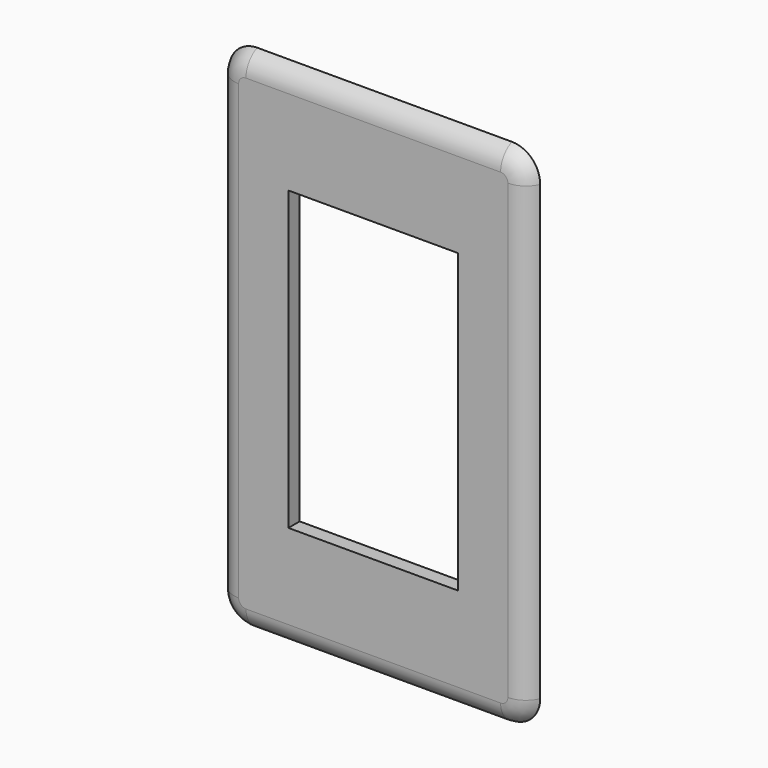
from build123d import *

# Parameters (mm, degrees)
F0_W         = 38.1
F0_H         = 66.675
F1_DEPTH     = 3.175
F2_T1_DEPTH  = 57.15
F2_T3_DEPTH  = 101.6
F2_T6_ANGLE  = 90
F2_T8_ANGLE  = 90
F2_T10_ANGLE = 90
F2_T12_ANGLE = 90


# Not quite as in the source:
# - a fillet or chamfer that OpenCascade refuses, or shapes differently, is made with other operations: its cross-section is extruded or revolved along the edge and cut away or added


with BuildPart() as f1:
    # F0 (on Front) → F1 (new body)
    with BuildSketch(Plane.XZ):
        with BuildLine():
            ThreePointArc((0, 6.35), (1.8598719395, 1.8598719395), (6.35, 0))
            Line((6.35, 0), (63.5, 0))
            ThreePointArc((63.5, 0), (67.9901280605, 1.8598719395), (69.85, 6.35))
            Line((69.85, 6.35), (69.85, 107.95))
            ThreePointArc((69.85, 107.95), (67.9901280605, 112.4401280605), (63.5, 114.3))
            Line((63.5, 114.3), (6.35, 114.3))
            ThreePointArc((6.35, 114.3), (1.8598719395, 112.4401280605), (0, 107.95))
            Line((0, 107.95), (0, 6.35))
        make_face()
        with Locations((34.925, 57.15)):
            Rectangle(F0_W, F0_H, mode=Mode.SUBTRACT)
    extrude(amount=F1_DEPTH)

    # F2: fillet of radius 5.08 on 1 edges, made by hand

    # F2_s2 → F2_t1 (cut)
    with BuildSketch(Plane.YZ.offset(6.35)):
        with BuildLine():
            ThreePointArc((0, 114.3), (-2.3071134838, 112.4305202921), (-3.175, 109.5907139607))
            Line((-3.175, 109.5907139607), (-3.175, 114.3))
            Line((-3.175, 114.3), (0, 114.3))
        make_face()
        with BuildLine():
            ThreePointArc((0, 0), (-2.3071134838, 1.8694797079), (-3.175, 4.7092860393))
            Line((-3.175, 4.7092860393), (-3.175, 0))
            Line((-3.175, 0), (0, 0))
        make_face()
    extrude(amount=F2_T1_DEPTH, mode=Mode.SUBTRACT)

    # F2_s4 → F2_t3 (cut)
    with BuildSketch(Plane.XY.offset(6.35)):
        with BuildLine():
            ThreePointArc((0, 0), (1.8694797079, -2.3071134838), (4.7092860393, -3.175))
            Line((4.7092860393, -3.175), (0, -3.175))
            Line((0, -3.175), (0, 0))
        make_face()
        with BuildLine():
            ThreePointArc((69.85, 0), (67.9805202921, -2.3071134838), (65.1407139607, -3.175))
            Line((65.1407139607, -3.175), (69.85, -3.175))
            Line((69.85, -3.175), (69.85, 0))
        make_face()
    extrude(amount=F2_T3_DEPTH, mode=Mode.SUBTRACT)

    # F2_s5 → F2_t6 (revolve, cut)
    with BuildSketch(Plane.XY.offset(107.95)):
        with BuildLine():
            ThreePointArc((69.85, 0), (67.9805202921, -2.3071134838), (65.1407139607, -3.175))
            Line((65.1407139607, -3.175), (69.85, -3.175))
            Line((69.85, -3.175), (69.85, 0))
        make_face()
    revolve(axis=Axis((63.5, -3.175, 107.95), (0, -1, 0)), revolution_arc=F2_T6_ANGLE, mode=Mode.SUBTRACT)

    # F2_s7 → F2_t8 (revolve, cut)
    with BuildSketch(Plane.YZ.offset(6.35)):
        with BuildLine():
            ThreePointArc((0, 114.3), (-2.3071134838, 112.4305202921), (-3.175, 109.5907139607))
            Line((-3.175, 109.5907139607), (-3.175, 114.3))
            Line((-3.175, 114.3), (0, 114.3))
        make_face()
    revolve(axis=Axis((6.35, -3.175, 107.95), (0, -1, 0)), revolution_arc=F2_T8_ANGLE, mode=Mode.SUBTRACT)

    # F2_s9 → F2_t10 (revolve, cut)
    with BuildSketch(Plane.XY.offset(6.35)):
        with BuildLine():
            ThreePointArc((0, 0), (1.8694797079, -2.3071134838), (4.7092860393, -3.175))
            Line((4.7092860393, -3.175), (0, -3.175))
            Line((0, -3.175), (0, 0))
        make_face()
    revolve(axis=Axis((6.35, -3.175, 6.35), (0, -1, 0)), revolution_arc=F2_T10_ANGLE, mode=Mode.SUBTRACT)

    # F2_s11 → F2_t12 (revolve, cut)
    with BuildSketch(Plane.YZ.offset(63.5)):
        with BuildLine():
            ThreePointArc((0, 0), (-2.3071134838, 1.8694797079), (-3.175, 4.7092860393))
            Line((-3.175, 4.7092860393), (-3.175, 0))
            Line((-3.175, 0), (0, 0))
        make_face()
    revolve(axis=Axis((63.5, -3.175, 6.35), (0, -1, 0)), revolution_arc=F2_T12_ANGLE, mode=Mode.SUBTRACT)


solid = f1.part
